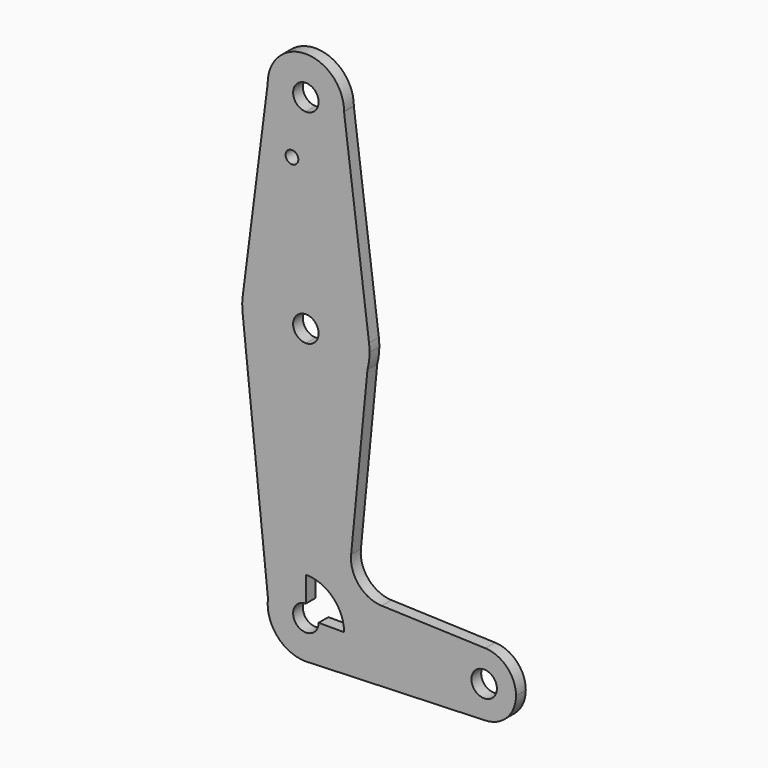
from build123d import *

# Parameters (mm, degrees)
F0_R     = 1.5875
F1_DEPTH = 3.048


# Not quite as in the source:
# - ends of sketch curves that miss each other by under 0.0002 mm in the source are joined


with BuildPart() as f1:
    # F0 (on Front) → F1 (new body)
    with BuildSketch(Plane.XZ):
        with BuildLine():
            ThreePointArc((-20.4063861121, 50.6759697353), (-20.4057804387, 50.7379835531), (-20.4055785447, 50.8))
            ThreePointArc((-20.4055785447, 50.8), (-29.9930844021, 60.3247949069), (-39.454758181, 50.6749909771))
            ThreePointArc((-39.454758181, 50.6749909771), (-36.6214272972, 44.0207546164), (-29.9305785447, 41.275))
            ThreePointArc((-29.9305785447, 41.275), (-23.2393814647, 44.0210984197), (-20.4063861121, 50.6759697353))
        make_face()
        with BuildLine():
            ThreePointArc((-26.7555785447, 50.8), (-27.6855145145, 48.5549359697), (-29.9305785447, 47.625))
            ThreePointArc((-29.9305785447, 47.625), (-32.175642575, 53.0450640303), (-26.7555785447, 50.8))
        make_face(mode=Mode.SUBTRACT)
        with BuildLine():
            ThreePointArc((-29.9305785447, 41.275), (-36.6214272972, 44.0207546164), (-39.454758181, 50.6749909771))
            Line((-39.454758181, 50.6749909771), (-45.6773538826, 2.0136264451))
            ThreePointArc((-45.6773538826, 2.0136264451), (-40.4198422268, 11.9159964924), (-29.9305785447, 15.875))
            Line((-29.9305785447, 15.875), (-29.9305785447, 41.275))
        make_face()
        with Locations((-33.3938002586, 36.5252)):
            Circle(F0_R, mode=Mode.SUBTRACT)
        with BuildLine():
            Line((-14.1837976059, 2.0135826444), (-20.4063861121, 50.6759697353))
            ThreePointArc((-20.4063861121, 50.6759697353), (-23.2393814647, 44.0210984197), (-29.9305785447, 41.275))
            Line((-29.9305785447, 41.275), (-29.9305785447, 15.875))
            ThreePointArc((-29.9305785447, 15.875), (-19.4412982901, 11.9159819041), (-14.1837976059, 2.0135826444))
        make_face()
        with BuildLine():
            ThreePointArc((-29.9305785447, 15.875), (-40.4198422268, 11.9159964924), (-45.6773538826, 2.0136264451))
            ThreePointArc((-45.6773538826, 2.0136264451), (-45.8043998708, -0.1934463924), (-45.6236065946, -2.3967677453))
            ThreePointArc((-45.6236065946, -2.3967677453), (-40.2738598675, -12.0429297298), (-29.9305785447, -15.875))
            Line((-29.9305785447, -15.875), (-29.9305785447, -3.175))
            ThreePointArc((-29.9305785447, -3.175), (-33.1055785447, 0), (-29.9305785447, 3.175))
            Line((-29.9305785447, 3.175), (-29.9305785447, 15.875))
        make_face()
        with BuildLine():
            ThreePointArc((-14.0555785447, 0), (-14.087665738, 1.0088304111), (-14.1837976059, 2.0135826444))
            ThreePointArc((-14.1837976059, 2.0135826444), (-19.4412982901, 11.9159819041), (-29.9305785447, 15.875))
            Line((-29.9305785447, 15.875), (-29.9305785447, 3.175))
            ThreePointArc((-29.9305785447, 3.175), (-27.6855145145, 2.2450640303), (-26.7555785447, 0))
            ThreePointArc((-26.7555785447, 0), (-27.6855145145, -2.2450640303), (-29.9305785447, -3.175))
            Line((-29.9305785447, -3.175), (-29.9305785447, -15.875))
            ThreePointArc((-29.9305785447, -15.875), (-20.2346648726, -12.5699993263), (-14.5759167084, -4.031127))
            ThreePointArc((-14.5759167084, -4.031127), (-14.1862004743, -2.0322854558), (-14.0555785447, 0))
        make_face()
        with BuildLine():
            ThreePointArc((-29.9305785447, -15.875), (-40.2738598675, -12.0429297298), (-45.6236065946, -2.3967677453))
            Line((-45.6236065946, -2.3967677453), (-39.3767361242, -62.2769987798))
            ThreePointArc((-39.3767361242, -62.2769987798), (-36.2185248858, -56.3454660661), (-29.9305785447, -53.975))
            Line((-29.9305785447, -53.975), (-29.9305785447, -15.875))
        make_face()
        with BuildLine():
            ThreePointArc((-14.5759167084, -4.031127), (-20.2346648726, -12.5699993263), (-29.9305785447, -15.875))
            Line((-29.9305785447, -15.875), (-29.9305785447, -53.975))
            ThreePointArc((-29.9305785447, -53.975), (-23.1953864539, -56.7648079092), (-20.4055785447, -63.5))
            Line((-20.4055785447, -63.5), (6.5819214553, -63.5))
            ThreePointArc((6.5819214553, -63.5), (9.0069371863, -57.7889209921), (14.8002328719, -55.5674688026))
            Line((14.8002328719, -55.5674688026), (-11.021864061, -54.648172114))
            ThreePointArc((-11.021864061, -54.648172114), (-16.7206173005, -51.9399910767), (-18.6518593628, -45.9333000481))
            Line((-18.6518593628, -45.9333000481), (-14.5759167084, -4.031127))
        make_face()
        with BuildLine():
            ThreePointArc((-29.9305785447, -53.975), (-36.2185248858, -56.3454660661), (-39.3767361242, -62.2769987798))
            ThreePointArc((-39.3767361242, -62.2769987798), (-37.1496877578, -69.7137015675), (-30.1273622995, -73.0229670352))
            Line((-30.1273622995, -73.0229670352), (-29.0609056002, -72.9852144925))
            ThreePointArc((-29.0609056002, -72.9852144925), (-22.8946258802, -69.920357864), (-20.4055785447, -63.5))
            Line((-20.4055785447, -63.5), (-26.7555785447, -63.5))
            ThreePointArc((-26.7555785447, -63.5), (-32.175642575, -65.7450640303), (-29.9305785447, -60.325))
            Line((-29.9305785447, -60.325), (-29.9305785447, -53.975))
        make_face()
        with BuildLine():
            Line((-29.0609056002, -72.9852144925), (-30.1273622995, -73.0229670352))
            ThreePointArc((-30.1273622995, -73.0229670352), (-29.593604838, -73.0190374367), (-29.0609056002, -72.9852144925))
        make_face()
        with BuildLine():
            Line((6.5819214553, -63.5), (-20.4055785447, -63.5))
            ThreePointArc((-20.4055785447, -63.5), (-22.8946258802, -69.920357864), (-29.0609056002, -72.9852144925))
            Line((-29.0609056002, -72.9852144925), (14.8002328776, -71.4325311972))
            ThreePointArc((14.8002328776, -71.4325311972), (9.0069371884, -69.2110790099), (6.5819214553, -63.5))
        make_face()
        with BuildLine():
            ThreePointArc((14.8002328719, -55.5674688026), (9.0069371863, -57.7889209921), (6.5819214553, -63.5))
            ThreePointArc((6.5819214553, -63.5), (9.0069371884, -69.2110790099), (14.8002328776, -71.4325311972))
            ThreePointArc((14.8002328776, -71.4325311972), (20.2305004652, -69.0124842669), (22.4569214553, -63.5))
            ThreePointArc((22.4569214553, -63.5), (20.2305004632, -57.9875157311), (14.8002328719, -55.5674688026))
        make_face()
        with BuildLine():
            ThreePointArc((17.6944214553, -63.5), (14.5194214553, -66.675), (11.3444214553, -63.5))
            ThreePointArc((11.3444214553, -63.5), (14.5194214553, -60.325), (17.6944214553, -63.5))
        make_face(mode=Mode.SUBTRACT)
    extrude(amount=F1_DEPTH)


solid = f1.part
